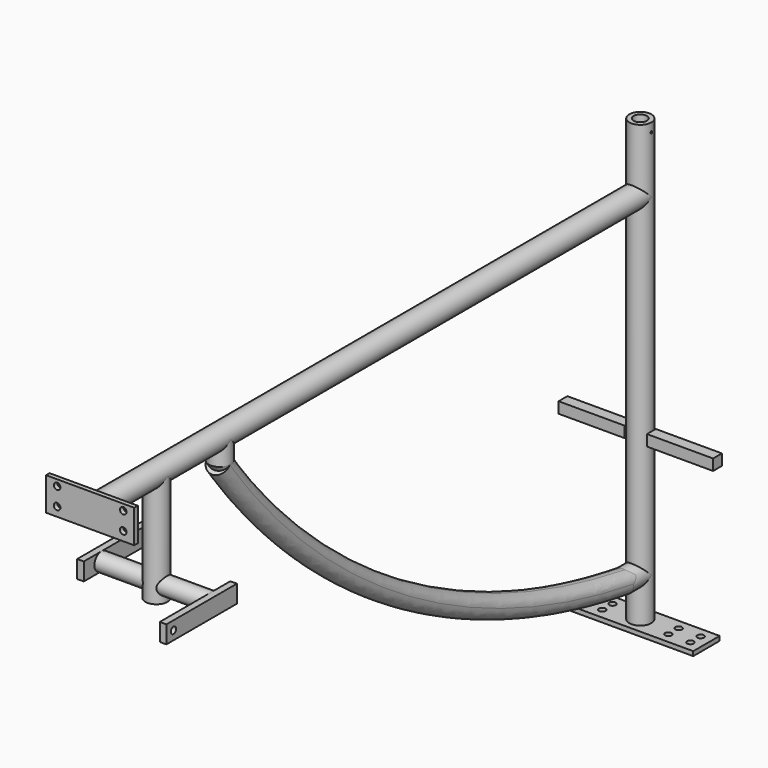
from build123d import *

# Parameters (mm, degrees)
F0_R      = 12.7
F0_R_2    = 7.62
F1_DEPTH  = 508
F2_R      = 12.7
F2_R_2    = 7.62
F3_DEPTH  = 787.4
F6_R      = 12.7
F8_DEPTH  = 25.4
F4_R      = 12.7
F9_DEPTH  = 25.4
F8_FACE_R = 12.7
F9_FACE_R = 12.7
F12_W     = 152.4
F12_H     = 38.1
F13_DEPTH = 5.08
F14_D     = 7.62
F17_W     = 12.7
F17_H     = 12.7
F18_DEPTH = 76.2
F22_W     = 12.7
F22_H     = 12.7
F23_DEPTH = 76.2
F27_D     = 2.54
F27_DEPTH = 76.201
F28_D     = 2.54
F31_R     = 12.7
F32_DEPTH = 127
F34_W     = 101.6
F34_H     = 38.1
F35_DEPTH = 5.08
F36_D     = 7.62
F38_D     = 20.32
F38_DEPTH = 76.201
F39_D     = 20.32
F39_DEPTH = 76.201
F37_R     = 10.16
F40_DEPTH = 63.5
F42_W     = 101.6
F42_H     = 20.32
F43_DEPTH = 7.62
F44_D     = 7.62
F47_DEPTH = 7.62
F48_D     = 7.62


# Not quite as in the source:
# - the program builds the solid bodies; features that only make, move or delete a surface that nothing else refers to are left out


with BuildPart() as f1:
    # F0 (on Top) → F1 (new body)
    with BuildSketch(Plane.XY):
        Circle(F0_R)
        Circle(F0_R_2, mode=Mode.SUBTRACT)
    extrude(amount=-F1_DEPTH)

    # F2 (on Front) → F3 (join)
    with BuildSketch(Plane.XZ):
        with Locations((0, -75.4170566797)):
            Circle(F2_R)
        with Locations((0, -75.4170566797)):
            Circle(F2_R_2, mode=Mode.SUBTRACT)
    extrude(amount=F3_DEPTH)

    # F6 (on face) → F8 (join)
    with BuildSketch(Plane(origin=(0, 0, -75.4170566797), x_dir=(1, 0, 0), z_dir=(0, 0, -1))):
        with Locations((0, 605.7751774788)):
            Circle(F6_R)
    extrude(amount=F8_DEPTH)

    # F4 (on Front) → F9 (join)
    with BuildSketch(Plane.XZ):
        with Locations((0, -459.2119753361)):
            Circle(F4_R)
    extrude(amount=F9_DEPTH)

    # F10: sweep along a path in F7
    with BuildLine(Plane.YZ) as f10_path:
        ThreePointArc((-608.006298542, -101.5726923943), (-352.2102236014, -338.255786488), (-25.3767501563, -459.2119753361))
    # F8_face (on face) + F9_face (on face) → F10 (sweep)
    with BuildSketch(Plane(origin=(0, -605.7751774788, -100.8170566797), x_dir=(1, 0, 0), z_dir=(0, 0, -1))):
        Circle(F8_FACE_R)
    with BuildSketch(Plane(origin=(0, -25.4, -459.2119753361), x_dir=(1, 0, 0), z_dir=(0, -1, 0))):
        Circle(F9_FACE_R)
    sweep(path=f10_path.line)

    # F12 (on offset) → F13 (join)
    with BuildSketch(Plane(origin=(0, 0, -508), x_dir=(1, 0, 0), z_dir=(0, 0, -1))):
        Rectangle(F12_W, F12_H)
    extrude(amount=F13_DEPTH)

    # F14 (through all)
    with Locations(Plane.XY.offset(-508)):
        with Locations((-63.5, -7.2122556157), (-63.5, 7.5626373291), (-38.1, 7.5626373291), (-38.1, -7.2122556157), (38.1, -7.2122556157), (38.1, 7.5626373291), (63.5, 7.5626373291), (63.5, -7.2122556157)):
            Hole(F14_D / 2)

    # F27 (through all, one way)
    with BuildSketch(Plane.YZ):
        with Locations((0, -10.1188989356)):
            Circle(F27_D / 2)
    extrude(amount=-F27_DEPTH, mode=Mode.SUBTRACT)

    # F28 (through all)
    with Locations(Plane(origin=(0, 0, 0), x_dir=(0, 1, 0), z_dir=(-1, 0, 0))):
        with Locations((0, 10.1188989356)):
            Hole(F28_D / 2)

    # F31 (on mid) → F32 (join)
    with BuildSketch(Plane(origin=(0, 0, -76.1171244085), x_dir=(1, 0, 0), z_dir=(0, 0, -1))):
        with Locations((0, 696.9612836838)):
            Circle(F31_R)
    extrude(amount=F32_DEPTH)

    # F34 (on offset) → F35 (join)
    with BuildSketch(Plane.XZ.offset(787.4)):
        with Locations((0, -75.4357725382)):
            Rectangle(F34_W, F34_H)
    extrude(amount=F35_DEPTH)

    # F36 (through all)
    with Locations(Plane(origin=(0, -787.4, 0), x_dir=(1, 0, 0), z_dir=(0, 1, 0))):
        with Locations((-38.1, 63.5107830167), (38.1, 63.5107830167), (38.1, 84.0243920684), (-38.1, 84.0243920684)):
            Hole(F36_D / 2)

    # F38 (through all, one way)
    with BuildSketch(Plane.YZ):
        with Locations((-696.9258189201, -186.6551935673)):
            Circle(F38_D / 2)
    extrude(amount=-F38_DEPTH, mode=Mode.SUBTRACT)

    # F39 (through all, one way)
    with BuildSketch(Plane(origin=(0, 0, 0), x_dir=(0, 1, 0), z_dir=(-1, 0, 0))):
        with Locations((-696.8464851379, 186.7036819458)):
            Circle(F39_D / 2)
    extrude(amount=-F39_DEPTH, mode=Mode.SUBTRACT)

    # F37 (on Right) → F40 (join, symmetric)
    with BuildSketch(Plane.YZ):
        with Locations((-696.8464851379, -186.7036819458)):
            Circle(F37_R)
    extrude(amount=F40_DEPTH, both=True)

    # F42 (on offset) → F43 (join)
    with BuildSketch(Plane.YZ.offset(63.5)):
        with Locations((-720.8084122658, -186.7253771687)):
            Rectangle(F42_W, F42_H)
    extrude(amount=F43_DEPTH)

    # F44 (through all)
    with Locations(Plane(origin=(63.5, 0, 0), x_dir=(0, 1, 0), z_dir=(-1, 0, 0))):
        with Locations((-761.4484122658, 186.7253771687)):
            Hole(F44_D / 2)

    # F46 (on offset) → F47 (join)
    with BuildSketch(Plane(origin=(-63.5, 0, 0), x_dir=(0, -1, 0), z_dir=(-1, 0, 0))):
        Polygon((722.3048976898, -176.5562129545), (696.9048976898, -176.5562129545), (620.7048976898, -176.5562129545), (620.7048976898, -196.8762129545), (696.9048976898, -196.8762129545), (722.3048976898, -196.8762129545), align=None)
    extrude(amount=F47_DEPTH)

    # F48 (through all)
    with Locations(Plane(origin=(-63.5, 0, 0), x_dir=(0, -1, 0), z_dir=(1, 0, 0))):
        with Locations((630.8648976898, 186.7162129545)):
            Hole(F48_D / 2)


with BuildPart() as f18:
    # F17 (on mid) → F18 (new body)
    with BuildSketch(Plane(origin=(12.7398534678, 0, 0), x_dir=(0, -1, 0), z_dir=(-1, 0, 0))):
        with Locations((0, -319.9060559273)):
            Rectangle(F17_W, F17_H)
    extrude(amount=-F18_DEPTH)


with BuildPart() as f23:
    # F22 (on mid) → F23 (new body)
    with BuildSketch(Plane.YZ.offset(-12.9624265246)):
        with Locations((0, -319.7445869446)):
            Rectangle(F22_W, F22_H)
    extrude(amount=-F23_DEPTH)


solid = Compound([f1.part, f18.part, f23.part])
